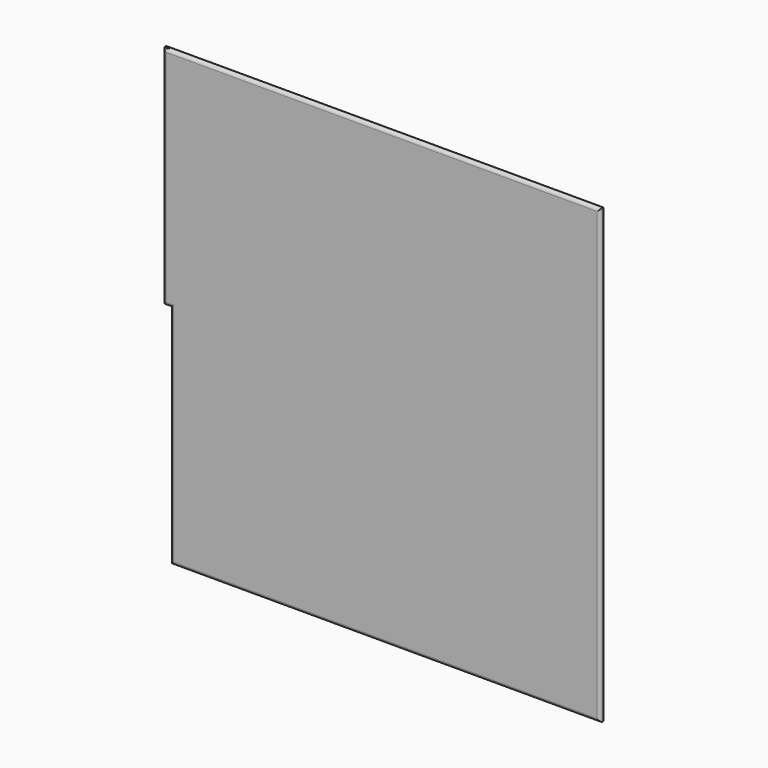
from build123d import *

# Parameters (mm, degrees)
F1_DEPTH     = 4
F2_R         = 1
F3_DEPTH     = 310
F4_T1_DEPTH  = 300
F4_T3_DEPTH  = 160
F4_T5_DEPTH  = 10
F4_T7_DEPTH  = 155
F4_T9_DEPTH  = 295
F4_T11_DEPTH = 310
F4_T17_DEPTH = 15
F4_T21_DEPTH = 160
F5_T1_DEPTH  = 300
F5_T3_DEPTH  = 160
F5_T5_DEPTH  = 10
F5_T7_DEPTH  = 155
F5_T9_DEPTH  = 295
F5_T11_DEPTH = 310
F5_T17_DEPTH = 15
F5_T21_DEPTH = 160


# Not quite as in the source:
# - a fillet or chamfer that OpenCascade refuses, or shapes differently, is made with other operations: its cross-section is extruded or revolved along the edge and cut away or added


with BuildPart() as f1:
    # F0 (on Front) → F1 (new body)
    with BuildSketch(Plane.XZ):
        Polygon((251.4121359825, 250.8489221025), (-38.5878640175, 250.8489221025), (-38.5878640175, 100.8489221025), (-33.5878640175, 100.8489221025), (-33.5878640175, -49.1510778975), (251.4121359825, -49.1510778975), align=None)
    extrude(amount=F1_DEPTH)

    # F2 (on face) → F3 (cut)
    with BuildSketch(Plane.XY.offset(250.8489221025)):
        with Locations((-36.5878640175, -2)):
            Circle(F2_R)
    extrude(amount=-F3_DEPTH, mode=Mode.SUBTRACT)

    # F4: fillet of radius 2 on 6 edges, made by hand

    # F4_s2 → F4_t1 (cut)
    with BuildSketch(Plane.YZ.offset(-43.5878640175)):
        with BuildLine():
            ThreePointArc((-2, 250.8489221025), (-3.4142135624, 250.2631356648), (-4, 248.8489221025))
            Line((-4, 248.8489221025), (-4, 250.8489221025))
            Line((-4, 250.8489221025), (-2, 250.8489221025))
        make_face()
    extrude(amount=F4_T1_DEPTH, mode=Mode.SUBTRACT)

    # F4_s4 → F4_t3 (cut)
    with BuildSketch(Plane.XY.offset(95.8489221025)):
        with BuildLine():
            ThreePointArc((-36.5878640175, -4), (-38.0020775799, -3.4142135624), (-38.5878640175, -2))
            Line((-38.5878640175, -2), (-38.5878640175, -4))
            Line((-38.5878640175, -4), (-36.5878640175, -4))
        make_face()
    extrude(amount=F4_T3_DEPTH, mode=Mode.SUBTRACT)

    # F4_s6 → F4_t5 (cut)
    with BuildSketch(Plane.YZ.offset(-43.5878640175)):
        with BuildLine():
            ThreePointArc((-4, 102.8489221025), (-3.4142135624, 101.4347085401), (-2, 100.8489221025))
            Line((-2, 100.8489221025), (-4, 100.8489221025))
            Line((-4, 100.8489221025), (-4, 102.8489221025))
        make_face()
    extrude(amount=F4_T5_DEPTH, mode=Mode.SUBTRACT)

    # F4_s8 → F4_t7 (cut)
    with BuildSketch(Plane.XY.offset(-54.1510778975)):
        with BuildLine():
            ThreePointArc((-31.5878640175, -4), (-33.0020775799, -3.4142135624), (-33.5878640175, -2))
            Line((-33.5878640175, -2), (-33.5878640175, -4))
            Line((-33.5878640175, -4), (-31.5878640175, -4))
        make_face()
    extrude(amount=F4_T7_DEPTH, mode=Mode.SUBTRACT)

    # F4_s10 → F4_t9 (cut)
    with BuildSketch(Plane.YZ.offset(-38.5878640175)):
        with BuildLine():
            ThreePointArc((-4, -47.1510778975), (-3.4142135624, -48.5652914599), (-2, -49.1510778975))
            Line((-2, -49.1510778975), (-4, -49.1510778975))
            Line((-4, -49.1510778975), (-4, -47.1510778975))
        make_face()
    extrude(amount=F4_T9_DEPTH, mode=Mode.SUBTRACT)

    # F4_s12 → F4_t11 (cut)
    with BuildSketch(Plane.XY.offset(-54.1510778975)):
        with BuildLine():
            ThreePointArc((251.4121359825, -2), (250.8263495449, -3.4142135624), (249.4121359825, -4))
            Line((249.4121359825, -4), (251.4121359825, -4))
            Line((251.4121359825, -4), (251.4121359825, -2))
        make_face()
    extrude(amount=F4_T11_DEPTH, mode=Mode.SUBTRACT)


with BuildPart() as f4_tool15:
    # F4_s16 → F4_t17 (new body)
    with BuildSketch(Plane.YZ.offset(-43.5878640175)):
        with BuildLine():
            ThreePointArc((-4, 102.8489221025), (-3.4142135624, 101.4347085401), (-2, 100.8489221025))
            Line((-2, 100.8489221025), (-4, 100.8489221025))
            Line((-4, 100.8489221025), (-4, 102.8489221025))
        make_face()
    extrude(amount=F4_T17_DEPTH)

    split(bisect_by=Plane.YZ.offset(-33.5878640175), keep=Keep.TOP)


with BuildPart() as f4_tool19:
    # F4_s20 → F4_t21 (new body)
    with BuildSketch(Plane.XY.offset(105.8489221025)):
        with BuildLine():
            ThreePointArc((-31.5878640175, -4), (-33.0020775799, -3.4142135624), (-33.5878640175, -2))
            Line((-33.5878640175, -2), (-33.5878640175, -4))
            Line((-33.5878640175, -4), (-31.5878640175, -4))
        make_face()
    extrude(amount=-F4_T21_DEPTH)

    split(bisect_by=Plane.XY.offset(100.8489221025), keep=Keep.TOP)


with BuildPart() as f4_tool15_1:
    add(f4_tool15.part)

    # F4_t23: intersect F4_tool19
    add(f4_tool19.part, mode=Mode.INTERSECT)


with BuildPart() as f1_1:
    add(f1.part)

    # F4_t13: cut F4_tool15
    add(f4_tool15_1.part, mode=Mode.SUBTRACT)

    # F5: fillet of radius 2 on 6 edges, made by hand

    # F5_s2 → F5_t1 (cut)
    with BuildSketch(Plane.YZ.offset(-43.5878640175)):
        with BuildLine():
            ThreePointArc((-2, 250.8489221025), (-0.5857864376, 250.2631356648), (0, 248.8489221025))
            Line((0, 248.8489221025), (0, 250.8489221025))
            Line((0, 250.8489221025), (-2, 250.8489221025))
        make_face()
    extrude(amount=F5_T1_DEPTH, mode=Mode.SUBTRACT)

    # F5_s4 → F5_t3 (cut)
    with BuildSketch(Plane.XY.offset(95.8489221025)):
        with BuildLine():
            ThreePointArc((-36.5878640175, 0), (-38.0020775799, -0.5857864376), (-38.5878640175, -2))
            Line((-38.5878640175, -2), (-38.5878640175, 0))
            Line((-38.5878640175, 0), (-36.5878640175, 0))
        make_face()
    extrude(amount=F5_T3_DEPTH, mode=Mode.SUBTRACT)

    # F5_s6 → F5_t5 (cut)
    with BuildSketch(Plane.YZ.offset(-43.5878640175)):
        with BuildLine():
            ThreePointArc((0, 102.8489221025), (-0.5857864376, 101.4347085401), (-2, 100.8489221025))
            Line((-2, 100.8489221025), (0, 100.8489221025))
            Line((0, 100.8489221025), (0, 102.8489221025))
        make_face()
    extrude(amount=F5_T5_DEPTH, mode=Mode.SUBTRACT)

    # F5_s8 → F5_t7 (cut)
    with BuildSketch(Plane.XY.offset(-54.1510778975)):
        with BuildLine():
            ThreePointArc((-31.5878640175, 0), (-33.0020775799, -0.5857864376), (-33.5878640175, -2))
            Line((-33.5878640175, -2), (-33.5878640175, 0))
            Line((-33.5878640175, 0), (-31.5878640175, 0))
        make_face()
    extrude(amount=F5_T7_DEPTH, mode=Mode.SUBTRACT)

    # F5_s10 → F5_t9 (cut)
    with BuildSketch(Plane.YZ.offset(-38.5878640175)):
        with BuildLine():
            ThreePointArc((0, -47.1510778975), (-0.5857864376, -48.5652914599), (-2, -49.1510778975))
            Line((-2, -49.1510778975), (0, -49.1510778975))
            Line((0, -49.1510778975), (0, -47.1510778975))
        make_face()
    extrude(amount=F5_T9_DEPTH, mode=Mode.SUBTRACT)

    # F5_s12 → F5_t11 (cut)
    with BuildSketch(Plane.XY.offset(-54.1510778975)):
        with BuildLine():
            ThreePointArc((249.4121359825, 0), (250.8263495449, -0.5857864376), (251.4121359825, -2))
            Line((251.4121359825, -2), (251.4121359825, 0))
            Line((251.4121359825, 0), (249.4121359825, 0))
        make_face()
    extrude(amount=F5_T11_DEPTH, mode=Mode.SUBTRACT)


with BuildPart() as f5_tool15:
    # F5_s16 → F5_t17 (new body)
    with BuildSketch(Plane.YZ.offset(-43.5878640175)):
        with BuildLine():
            ThreePointArc((0, 102.8489221025), (-0.5857864376, 101.4347085401), (-2, 100.8489221025))
            Line((-2, 100.8489221025), (0, 100.8489221025))
            Line((0, 100.8489221025), (0, 102.8489221025))
        make_face()
    extrude(amount=F5_T17_DEPTH)

    split(bisect_by=Plane.YZ.offset(-33.5878640175), keep=Keep.TOP)


with BuildPart() as f5_tool19:
    # F5_s20 → F5_t21 (new body)
    with BuildSketch(Plane.XY.offset(105.8489221025)):
        with BuildLine():
            ThreePointArc((-31.5878640175, 0), (-33.0020775799, -0.5857864376), (-33.5878640175, -2))
            Line((-33.5878640175, -2), (-33.5878640175, 0))
            Line((-33.5878640175, 0), (-31.5878640175, 0))
        make_face()
    extrude(amount=-F5_T21_DEPTH)

    split(bisect_by=Plane.XY.offset(100.8489221025), keep=Keep.TOP)


with BuildPart() as f5_tool15_1:
    add(f5_tool15.part)

    # F5_t23: intersect F5_tool19
    add(f5_tool19.part, mode=Mode.INTERSECT)


with BuildPart() as f1_2:
    add(f1_1.part)

    # F5_t13: cut F5_tool15
    add(f5_tool15_1.part, mode=Mode.SUBTRACT)


solid = f1_2.part
